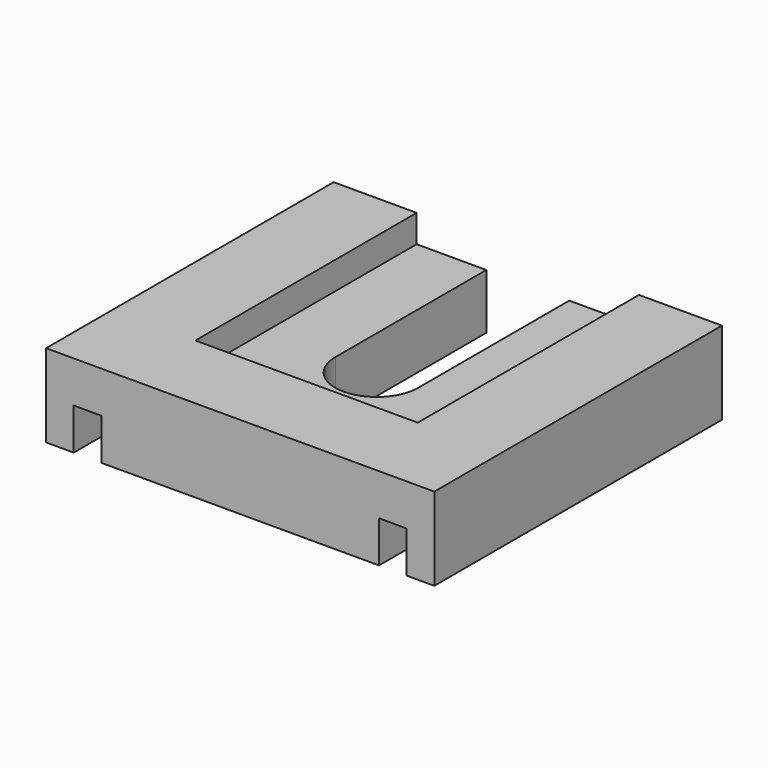
from build123d import *

# Parameters (mm, degrees)
F1_DEPTH = 15
F2_DEPTH = 10
F3_W     = 2.5
F3_H     = 65
F4_DEPTH = 7.5


with BuildPart() as f1:
    # F0 (on Top) → F1 (new body)
    with BuildSketch(Plane.XY):
        Polygon((-34.4940570078, 34.1372138634), (-49.4940570078, 34.1372138634), (-49.4940570078, -30.8627861366), (20.7059429922, -30.8627861366), (20.7059429922, 34.1372138634), (5.7059429922, 34.1372138634), (5.7059429922, -15.8627861366), (-34.4940570078, -15.8627861366), align=None)
    extrude(amount=F1_DEPTH)

    # F0 (on Top) → F2 (join)
    with BuildSketch(Plane.XY):
        Polygon((-34.4940570078, 34.1372138634), (-49.4940570078, 34.1372138634), (-49.4940570078, -30.8627861366), (20.7059429922, -30.8627861366), (20.7059429922, 34.1372138634), (5.7059429922, 34.1372138634), (5.7059429922, -15.8627861366), (-34.4940570078, -15.8627861366), align=None)
        with BuildLine():
            Line((-21.8940570078, 34.1372138634), (-34.4940570078, 34.1372138634))
            Line((-34.4940570078, 34.1372138634), (-34.4940570078, -15.8627861366))
            Line((-34.4940570078, -15.8627861366), (5.7059429922, -15.8627861366))
            Line((5.7059429922, -15.8627861366), (5.7059429922, 34.1372138634))
            Line((5.7059429922, 34.1372138634), (-6.8940570078, 34.1372138634))
            Line((-6.8940570078, 34.1372138634), (-6.8940570078, 0))
            ThreePointArc((-6.8940570078, 0), (-14.3940570078, -7.5), (-21.8940570078, 0))
            Line((-21.8940570078, 0), (-21.8940570078, 34.1372138634))
        make_face()
    extrude(amount=F2_DEPTH)

    # F3 (on face) → F4 (cut, symmetric)
    with BuildSketch(Plane.XY):
        with Locations((-43.2440570078, 1.6372138634)):
            Rectangle(F3_W, F3_H)
        with Locations((-40.7440570078, 1.6372138634)):
            Rectangle(F3_W, F3_H)
        with BuildLine():
            Line((10.7059429922, 34.05405581), (10.7059429922, -30.8627861366))
            Line((10.7059429922, -30.8627861366), (13.2059429922, -30.8627861366))
            Line((13.2059429922, -30.8627861366), (15.7059429922, -30.8627861366))
            Line((15.7059429922, -30.8627861366), (15.7059429922, 34.05405581))
            ThreePointArc((15.7059429922, 34.05405581), (15.7055971095, 34.0956405901), (15.7045595571, 34.1372138634))
            Line((15.7045595571, 34.1372138634), (10.7073264274, 34.1372138634))
            ThreePointArc((10.7073264274, 34.1372138634), (10.7062888749, 34.0956405901), (10.7059429922, 34.05405581))
        make_face()
    extrude(amount=F4_DEPTH, both=True, mode=Mode.SUBTRACT)


solid = f1.part
